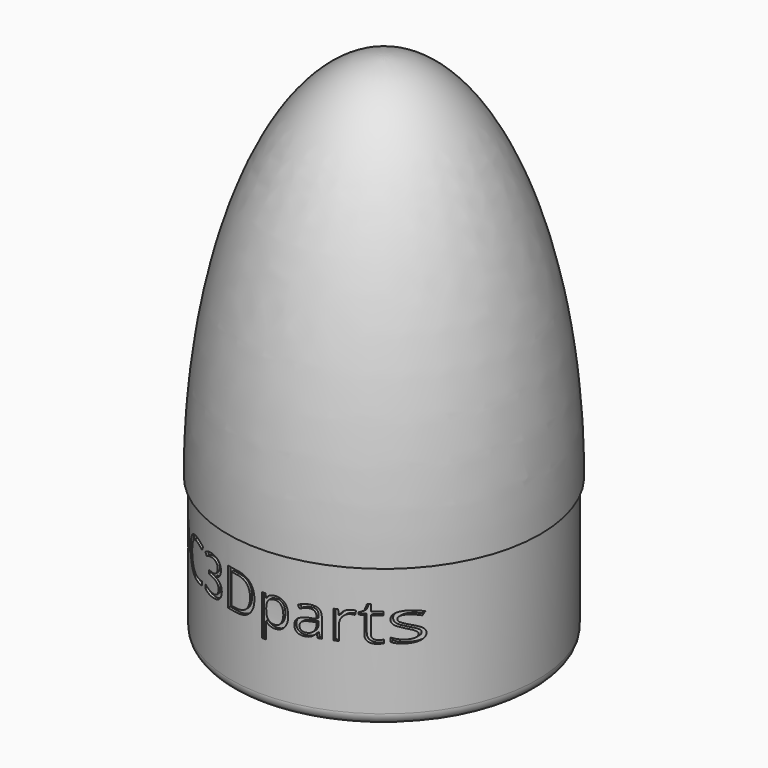
from build123d import *

# Parameters (mm, degrees)
F2_R         = 2.5
F5_W         = 32
F5_H         = 15.6837885009
F4_TEXT_SIZE = 11.1111111111
F7_DEPTH     = 40


# Not quite as in the source:
# - Text() gives the source's letters only with a copy of the font that has no kerning and outlines rounded to 1/6400 em; it was checked with that copy


with BuildPart() as f1:
    # F0 (on Front) → F1 (revolve)
    with BuildSketch(Plane.XZ):
        with BuildLine():
            Line((0, 0), (0, 78.7014423827))
            add(Edge.make_bspline(
                [(0, 78.7014423827), (-33.25, 78.7014423827), (-33.25, 0)],
                knots=[0, 0, 0, 1.5707963268, 1.5707963268, 1.5707963268], degree=2, weights=[1, 0.7071067812, 1]))
            Line((-33.25, 0), (-32.55, 0))
            Line((-32.55, 0), (-32.55, -30))
            Line((-32.55, -30), (0, -30))
            Line((0, -30), (0, 0))
        make_face()
    revolve(axis=Axis((0, 0, 1.4177560806), (0, 0, -1)))

    # F2
    f2_edges = [f1.edges().sort_by_distance(p)[0] for p in [
        (32.55, 0, -30),
    ]]
    fillet(f2_edges, radius=F2_R)


with BuildPart() as f6:
    # F5 (on Front) → F6 (revolve)
    with BuildSketch(Plane.XZ):
        with Locations((-16, -10.6906957552)):
            Rectangle(F5_W, F5_H)
    revolve(axis=Axis((0, 0, 1.4177560806), (0, 0, -1)))


with BuildPart() as f7:
    # F4 (on offset) → F7 (new body, through all)
    with BuildSketch(Plane.XZ.offset(40)):
        with Locations((-30.4371707735, -14.3152341657)):
            Text('DC3Dparts', F4_TEXT_SIZE, font='Open Sans', text_align=(TextAlign.LEFT, TextAlign.BOTTOM))
    extrude(amount=-F7_DEPTH)

    # F8: cut F6
    add(f6.part, mode=Mode.SUBTRACT)


with BuildPart() as f1_1:
    add(f1.part)

    # F9: cut F7
    add(f7.part, mode=Mode.SUBTRACT)


solid = f1_1.part
